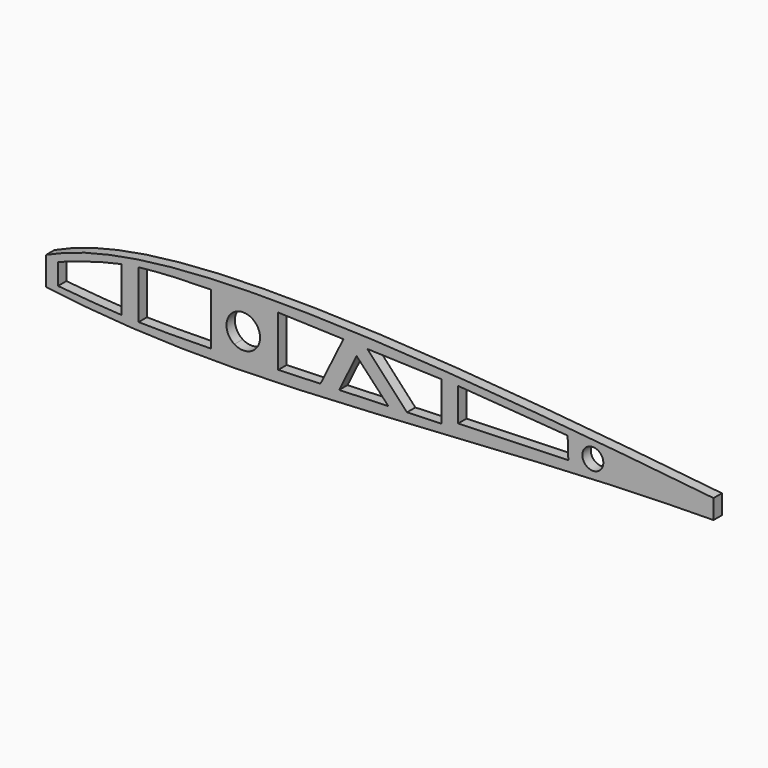
from build123d import *

# Parameters (mm, degrees)
F2_DEPTH = 2.5
F1_R     = 2.5
F3_DEPTH = 2.5
F5_DEPTH = 2.5
F6_DEPTH = 2.5
F7_DEPTH = 2.5
F8_DEPTH = 2.5
F9_DEPTH = 2.5


# Not quite as in the source:
# - a feature names something its author has since deleted; it is built from what else it names


with BuildPart() as f2:
    # F0 (on Front) → F2 (new body)
    with BuildSketch(Plane.XZ):
        with BuildLine():
            add(Edge.make_bspline(
                [(-96.9805282175, -0.8100506688), (-84.7869920978, 5.1468541776), (-38.6381415733, 10.9636146396), (42.6881882799, 2.4723259958), (100, -4.047003109)],
                knots=[0, 0, 0, 0, 0.374886421, 1, 1, 1, 1], degree=3))
            add(Edge.make_bspline(
                [(-97.5447368223, -7.1186651935), (-99.939251346, -6.5508492693), (-102.885147974, -5.168950634), (-100.0067471137, -2.3789404522), (-96.9805282175, -0.8100506688)],
                knots=[0.0564585679, 0.0564585679, 0.0564585679, 0.0564585679, 0.4847104148, 1, 1, 1, 1], degree=3))
            add(Edge.make_bspline(
                [(-96.5428845142, -7.3406707446), (-96.8949965543, -7.2673488468), (-97.22905608, -7.1935231869), (-97.5447368223, -7.1186651935)],
                knots=[0, 0, 0, 0, 0.0564585679, 0.0564585679, 0.0564585679, 0.0564585679], degree=3))
            add(Edge.make_bspline(
                [(-96.5428845142, -7.3406707446), (-80.7020161693, -9.4302402111), (-44.2471235075, -11.1181020976), (41.8622965332, -3.5518856086), (82.0915186506, -4.6802794425), (100, -4.047003109)],
                knots=[0, 0, 0, 0, 0.2987594418, 0.6837410955, 1, 1, 1, 1], degree=3))
        make_face()
        with BuildLine():
            add(Edge.make_bspline(
                [(-99.8196757147, -4.047003109), (-99.3821638101, -3.2227137691), (-97.9006497107, -2.3042858417), (-96.3385477662, -1.6362179573)],
                knots=[0.5425000514, 0.5425000514, 0.5425000514, 0.5425000514, 1, 1, 1, 1], degree=3))
            add(Edge.make_bspline(
                [(-96.3385477662, -1.6362179573), (-85.7442874691, 3.2900694446), (-38.7960585931, 10.0747672146), (36.943279708, 1.696590452), (86.094097513, -3.3751911245)],
                knots=[0, 0, 0, 0, 0.384923117, 1, 1, 1, 1], degree=3))
            add(Edge.make_bspline(
                [(-97.3825784566, -6.0471531808), (-82.3468325761, -8.841713568), (-44.2551066449, -8.6286827794), (40.9195716837, -3.3120714751), (72.7341022162, -3.1550192186), (86.094097513, -3.3751911245)],
                knots=[0, 0, 0, 0, 0.3131273629, 0.7122131732, 1, 1, 1, 1], degree=3))
            add(Edge.make_bspline(
                [(-97.3825784566, -6.0471531808), (-98.6588937786, -5.8946130057), (-100.1661659123, -5.1778479876), (-99.9138553768, -4.2244412327), (-99.8196757147, -4.047003109)],
                knots=[0, 0, 0, 0, 0.4440177242, 0.5425000514, 0.5425000514, 0.5425000514, 0.5425000514], degree=3))
        make_face(mode=Mode.SUBTRACT)
        with BuildLine():
            add(Edge.make_bspline(
                [(-96.3385477662, -1.6362179573), (-85.7442874691, 3.2900694446), (-38.7960585931, 10.0747672146), (36.943279708, 1.696590452), (86.094097513, -3.3751911245)],
                knots=[0, 0, 0, 0, 0.384923117, 1, 1, 1, 1], degree=3))
            add(Edge.make_bspline(
                [(-99.8196757147, -4.047003109), (-99.3821638101, -3.2227137691), (-97.9006497107, -2.3042858417), (-96.3385477662, -1.6362179573)],
                knots=[0.5425000514, 0.5425000514, 0.5425000514, 0.5425000514, 1, 1, 1, 1], degree=3))
            add(Edge.make_bspline(
                [(-97.3825784566, -6.0471531808), (-98.6588937786, -5.8946130057), (-100.1661659123, -5.1778479876), (-99.9138553768, -4.2244412327), (-99.8196757147, -4.047003109)],
                knots=[0, 0, 0, 0, 0.4440177242, 0.5425000514, 0.5425000514, 0.5425000514, 0.5425000514], degree=3))
            add(Edge.make_bspline(
                [(-97.3825784566, -6.0471531808), (-82.3468325761, -8.841713568), (-44.2551066449, -8.6286827794), (40.9195716837, -3.3120714751), (72.7341022162, -3.1550192186), (86.094097513, -3.3751911245)],
                knots=[0, 0, 0, 0, 0.3131273629, 0.7122131732, 1, 1, 1, 1], degree=3))
        make_face()
        with BuildLine():
            add(Edge.make_bspline(
                [(-96.5428845142, -7.3406707446), (-96.8949965543, -7.2673488468), (-97.22905608, -7.1935231869), (-97.5447368223, -7.1186651935)],
                knots=[0, 0, 0, 0, 0.0564585679, 0.0564585679, 0.0564585679, 0.0564585679], degree=3))
            ThreePointArc((-97.5447368223, -7.1186651935), (-97.052492706, -7.2688477084), (-96.5428845142, -7.3406707446))
        make_face()
    extrude(amount=F2_DEPTH)


with BuildPart() as f2b:
    # F1 (on Front) → F2, piece 2 (new body)
    with BuildSketch(Plane.XZ):
        with Locations((33.7789729238, -1.0305350879)):
            Circle(F1_R)
    extrude(amount=F2_DEPTH)


with BuildPart() as f2c:
    # F1 (on Front) → F2, piece 3 (new body)
    with BuildSketch(Plane.XZ):
        with BuildLine():
            ThreePointArc((-45.542362095, -1.3708024857), (-51.4789804014, 2.1291274472), (-51.6671168627, -4.7598166753))
            Line((-51.6671168627, -4.7598166753), (-47.385046135, -4.7391830831))
            ThreePointArc((-47.385046135, -4.7391830831), (-46.0331411102, -3.2905337378), (-45.542362095, -1.3708024857))
        make_face()
        with BuildLine():
            Line((-47.385046135, -4.7391830831), (-51.6671168627, -4.7598166753))
            ThreePointArc((-51.6671168627, -4.7598166753), (-49.523087913, -5.3707560487), (-47.385046135, -4.7391830831))
        make_face()
    extrude(amount=F2_DEPTH)


with BuildPart() as f3_tool:
    # F1 (on Front) → F3 (new body)
    with BuildSketch(Plane.XZ):
        with BuildLine():
            ThreePointArc((-45.542362095, -1.3708024857), (-51.4789804014, 2.1291274472), (-51.6671168627, -4.7598166753))
            Line((-51.6671168627, -4.7598166753), (-47.385046135, -4.7391830831))
            ThreePointArc((-47.385046135, -4.7391830831), (-46.0331411102, -3.2905337378), (-45.542362095, -1.3708024857))
        make_face()
        with BuildLine():
            Line((-47.385046135, -4.7391830831), (-51.6671168627, -4.7598166753))
            ThreePointArc((-51.6671168627, -4.7598166753), (-49.523087913, -5.3707560487), (-47.385046135, -4.7391830831))
        make_face()
        with Locations((33.7789729238, -1.0305350879)):
            Circle(F1_R)
    extrude(amount=F3_DEPTH)


with BuildPart() as f2_1:
    add(f2.part)

    # F3: cut by f3_tool
    add(f3_tool.part, mode=Mode.SUBTRACT)

    # F4 (on face) → F5 (cut)
    with BuildSketch(Plane.XZ.offset(2.5)):
        with BuildLine():
            Line((-96.5428845142, -7.3406707446), (-96.5428845142, -0.5989118026))
            add(Edge.make_bspline(
                [(-96.9805282175, -0.8100506688), (-96.8353706427, -0.7391368787), (-96.6894893165, -0.6687582494), (-96.5428845142, -0.5989118026)],
                knots=[0, 0, 0, 0, 0.0044628238, 0.0044628238, 0.0044628238, 0.0044628238], degree=3))
            add(Edge.make_bspline(
                [(-96.9805282175, -0.8100506688), (-100.0067471137, -2.3789404522), (-102.885147974, -5.168950634), (-99.939251346, -6.5508492693), (-97.5447368223, -7.1186651935)],
                knots=[0.0564585679, 0.0564585679, 0.0564585679, 0.0564585679, 0.5717481532, 1, 1, 1, 1], degree=3))
            ThreePointArc((-97.5447368223, -7.1186651935), (-97.052492706, -7.2688477084), (-96.5428845142, -7.3406707446))
        make_face()
    extrude(amount=-F5_DEPTH, mode=Mode.SUBTRACT)

    # F4 (on face) → F6 (cut)
    with BuildSketch(Plane.XZ.offset(2.5)):
        with BuildLine():
            Line((-78.6215588156, -7.3670944992), (-78.6215588156, 3.2958948603))
            add(Edge.make_bspline(
                [(-78.6215588156, 3.2958948603), (-83.9345486349, 2.2532028855), (-88.8194569144, 0.5548157735), (-93.7043651938, -1.1435713386)],
                knots=[0.554896308, 0.554896308, 0.554896308, 0.554896308, 1, 1, 1, 1], degree=3))
            Line((-93.7043651938, -1.1435713386), (-93.7043651938, -6.1954581179))
            add(Edge.make_bspline(
                [(-78.6215588156, -7.3670944992), (-83.7013643272, -7.1077100258), (-88.7028647605, -6.6515840718), (-93.7043651938, -6.1954581179)],
                knots=[0.5793594661, 0.5793594661, 0.5793594661, 0.5793594661, 1, 1, 1, 1], degree=3))
        make_face()
        with BuildLine():
            Line((-57.251535356, -7.4831936508), (-57.251535356, 4.8988820054))
            add(Edge.make_bspline(
                [(-57.251535356, 4.8988820054), (-63.1249518816, 4.7812850577), (-68.9983684072, 4.66368811), (-74.4892291338, 3.9601280834)],
                knots=[0, 0, 0, 0, 0.4418705618, 0.4418705618, 0.4418705618, 0.4418705618], degree=3))
            Line((-74.4892291338, 3.9601280834), (-74.4892291338, -7.5306241193))
            add(Edge.make_bspline(
                [(-57.251535356, -7.4831936508), (-63.0319736557, -7.5857864832), (-68.8124119553, -7.6883793156), (-74.4892291338, -7.5306241193)],
                knots=[0, 0, 0, 0, 0.4658094847, 0.4658094847, 0.4658094847, 0.4658094847], degree=3))
        make_face()
        Polygon((27.7735989974, 1.9125135442), (1.6607665457, 3.840460399), (1.6607665457, -4.047003109), (27.9367215699, -3.2103169474), align=None)
    extrude(amount=-F6_DEPTH, mode=Mode.SUBTRACT)

    # F4 (on face) → F7 (cut)
    with BuildSketch(Plane.XZ.offset(2.5)):
        with BuildLine():
            add(Edge.make_bspline(
                [(62.5460875734, 0.1020588345), (74.6514883615, -1.1873862537), (87.1633646635, -2.586811085), (100, -4.047003109)],
                knots=[0.8599877614, 0.8599877614, 0.8599877614, 0.8599877614, 1, 1, 1, 1], degree=3))
            Line((62.5460875734, 0.1020588345), (62.5460875734, -4.518638291))
            add(Edge.make_bspline(
                [(62.5460875734, -4.518638291), (75.9097127299, -4.3829595873), (88.0075171585, -4.4710790211), (100, -4.047003109)],
                knots=[0.7882160183, 0.7882160183, 0.7882160183, 0.7882160183, 1, 1, 1, 1], degree=3))
        make_face()
    extrude(amount=-F7_DEPTH, mode=Mode.SUBTRACT)

    # F4 (on face) → F8 (cut)
    with BuildSketch(Plane.XZ.offset(2.5)):
        with BuildLine():
            Line((-78.6215588156, -7.3670944992), (-78.6215588156, 3.2958948603))
            add(Edge.make_bspline(
                [(-78.6215588156, 3.2958948603), (-83.9345486349, 2.2532028855), (-88.8194569144, 0.5548157735), (-93.7043651938, -1.1435713386)],
                knots=[0.554896308, 0.554896308, 0.554896308, 0.554896308, 1, 1, 1, 1], degree=3))
            Line((-93.7043651938, -1.1435713386), (-93.7043651938, -6.1954581179))
            add(Edge.make_bspline(
                [(-78.6215588156, -7.3670944992), (-83.7013643272, -7.1077100258), (-88.7028647605, -6.6515840718), (-93.7043651938, -6.1954581179)],
                knots=[0.5793594661, 0.5793594661, 0.5793594661, 0.5793594661, 1, 1, 1, 1], degree=3))
        make_face()
        with BuildLine():
            Line((-57.251535356, -7.4831936508), (-57.251535356, 4.8988820054))
            add(Edge.make_bspline(
                [(-57.251535356, 4.8988820054), (-63.1249518816, 4.7812850577), (-68.9983684072, 4.66368811), (-74.4892291338, 3.9601280834)],
                knots=[0, 0, 0, 0, 0.4418705618, 0.4418705618, 0.4418705618, 0.4418705618], degree=3))
            Line((-74.4892291338, 3.9601280834), (-74.4892291338, -7.5306241193))
            add(Edge.make_bspline(
                [(-57.251535356, -7.4831936508), (-63.0319736557, -7.5857864832), (-68.8124119553, -7.6883793156), (-74.4892291338, -7.5306241193)],
                knots=[0, 0, 0, 0, 0.4658094847, 0.4658094847, 0.4658094847, 0.4658094847], degree=3))
        make_face()
        Polygon((-41.2043631077, 5.3020771593), (-41.2043631077, -6.7306268347), (-31.1431517353, -6.3803097993), (-25.6712666077, 4.7633535934), align=None)
        Polygon((27.7735989974, 1.9125135442), (1.6607665457, 3.840460399), (1.6607665457, -4.047003109), (27.9367215699, -3.2103169474), align=None)
    extrude(amount=-F8_DEPTH, mode=Mode.SUBTRACT)

    # F4 (on face) → F9 (cut)
    with BuildSketch(Plane.XZ.offset(2.5)):
        Polygon((-22.5247312337, 2.2527640685), (-26.6876633679, -6.2251760467), (-14.952923861, -5.8165891476), align=None)
        Polygon((-2.2568607237, 3.9512880641), (-19.9629371484, 4.5653755791), (-10.5242531862, -5.6623891488), (-2.2568607237, -5.3745303303), align=None)
        Polygon((27.7735989974, 1.9125135442), (1.6607665457, 3.840460399), (1.6607665457, -4.047003109), (27.9367215699, -3.2103169474), align=None)
        with BuildLine():
            Line((-57.251535356, -7.4831936508), (-57.251535356, 4.8988820054))
            add(Edge.make_bspline(
                [(-57.251535356, 4.8988820054), (-63.1249518816, 4.7812850577), (-68.9983684072, 4.66368811), (-74.4892291338, 3.9601280834)],
                knots=[0, 0, 0, 0, 0.4418705618, 0.4418705618, 0.4418705618, 0.4418705618], degree=3))
            Line((-74.4892291338, 3.9601280834), (-74.4892291338, -7.5306241193))
            add(Edge.make_bspline(
                [(-57.251535356, -7.4831936508), (-63.0319736557, -7.5857864832), (-68.8124119553, -7.6883793156), (-74.4892291338, -7.5306241193)],
                knots=[0, 0, 0, 0, 0.4658094847, 0.4658094847, 0.4658094847, 0.4658094847], degree=3))
        make_face()
        with BuildLine():
            Line((-78.6215588156, -7.3670944992), (-78.6215588156, 3.2958948603))
            add(Edge.make_bspline(
                [(-78.6215588156, 3.2958948603), (-83.9345486349, 2.2532028855), (-88.8194569144, 0.5548157735), (-93.7043651938, -1.1435713386)],
                knots=[0.554896308, 0.554896308, 0.554896308, 0.554896308, 1, 1, 1, 1], degree=3))
            Line((-93.7043651938, -1.1435713386), (-93.7043651938, -6.1954581179))
            add(Edge.make_bspline(
                [(-78.6215588156, -7.3670944992), (-83.7013643272, -7.1077100258), (-88.7028647605, -6.6515840718), (-93.7043651938, -6.1954581179)],
                knots=[0.5793594661, 0.5793594661, 0.5793594661, 0.5793594661, 1, 1, 1, 1], degree=3))
        make_face()
        Polygon((-41.2043631077, 5.3020771593), (-41.2043631077, -6.7306268347), (-31.1431517353, -6.3803097993), (-25.6712666077, 4.7633535934), align=None)
    extrude(amount=-F9_DEPTH, mode=Mode.SUBTRACT)


with BuildPart() as f2b_1:
    add(f2b.part)

    # F3: cut by f3_tool
    add(f3_tool.part, mode=Mode.SUBTRACT)


with BuildPart() as f2c_1:
    add(f2c.part)

    # F3: cut by f3_tool
    add(f3_tool.part, mode=Mode.SUBTRACT)


solid = f2_1.part
